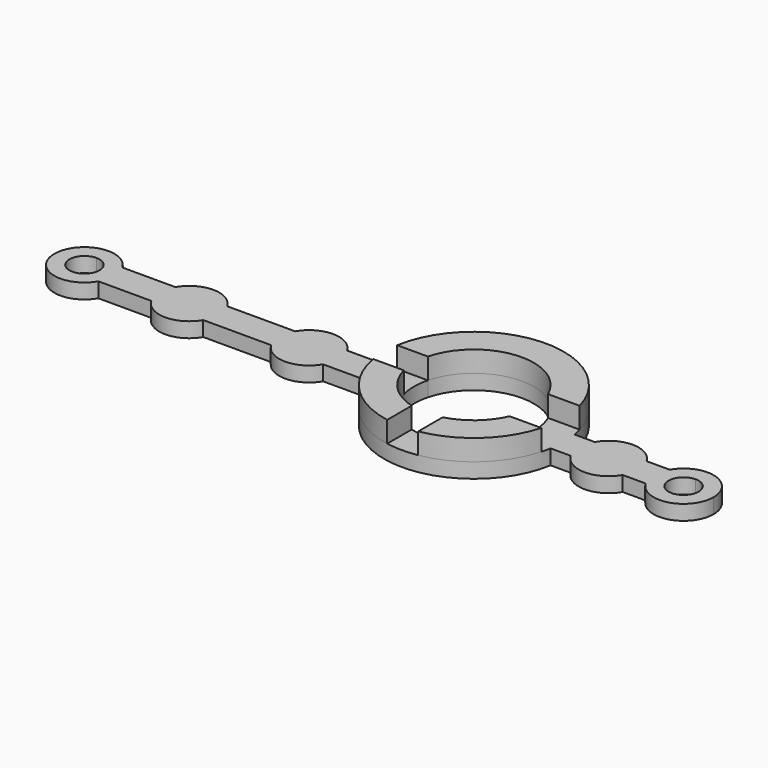
from build123d import *
from build123d import SkipClean  # not in build123d's __all__

# Parameters (mm, degrees)
F1_DEPTH = 5
F3_DEPTH = 7


with BuildPart() as f1:
    # F0 (on Top) → F1 (new body)
    with BuildSketch(Plane.XY):
        with BuildLine():
            ThreePointArc((0, 5), (3.5355339059, 3.5355339059), (5, 0))
            ThreePointArc((5, 0), (3.5355339059, -3.5355339059), (0, -5))
            Line((0, -5), (-8.6602540378, -5))
            ThreePointArc((-8.6602540378, -5), (2.588190451, -9.6592582629), (10, 0))
            ThreePointArc((10, 0), (2.588190451, 9.6592582629), (-8.6602540378, 5))
            Line((-8.6602540378, 5), (0, 5))
        make_face()
        with BuildLine():
            ThreePointArc((0, -5), (-5, 0), (0, 5))
            Line((0, 5), (-8.6602540378, 5))
            ThreePointArc((-8.6602540378, 5), (-10, 0), (-8.6602540378, -5))
            Line((-8.6602540378, -5), (0, -5))
        make_face()
        with BuildLine():
            ThreePointArc((-8.6602540378, -5), (-10, 0), (-8.6602540378, 5))
            Line((-8.6602540378, 5), (-16.3397459622, 5))
            ThreePointArc((-16.3397459622, 5), (-15.3407417371, 2.588190451), (-15, 0))
            ThreePointArc((-15, 0), (-15.3407417371, -2.588190451), (-16.3397459622, -5))
            Line((-16.3397459622, -5), (-8.6602540378, -5))
        make_face()
        with BuildLine():
            ThreePointArc((-15, 0), (-15.3407417371, 2.588190451), (-16.3397459622, 5))
            Line((-16.3397459622, 5), (-33.6602540378, 5))
            ThreePointArc((-33.6602540378, 5), (-35, 0), (-33.6602540378, -5))
            Line((-33.6602540378, -5), (-16.3397459622, -5))
            ThreePointArc((-16.3397459622, -5), (-15.3407417371, -2.588190451), (-15, 0))
        make_face()
        with BuildLine():
            Line((-33.6602540378, 5), (-16.3397459622, 5))
            ThreePointArc((-16.3397459622, 5), (-25, 10), (-33.6602540378, 5))
        make_face()
        with BuildLine():
            ThreePointArc((-33.6602540378, -5), (-25, -10), (-16.3397459622, -5))
            Line((-16.3397459622, -5), (-33.6602540378, -5))
        make_face()
        with BuildLine():
            ThreePointArc((-33.6602540378, -5), (-35, 0), (-33.6602540378, 5))
            Line((-33.6602540378, 5), (-40.4196010845, 5))
            ThreePointArc((-40.4196010845, 5), (-40.1050843164, 2.5087878084), (-40, 0))
            ThreePointArc((-40, 0), (-40.1050843164, -2.5087878084), (-40.4196010845, -5))
            Line((-40.4196010845, -5), (-33.6602540378, -5))
        make_face()
        with BuildLine():
            ThreePointArc((-40, 0), (-40.1050843164, 2.5087878084), (-40.4196010845, 5))
            Line((-40.4196010845, 5), (-50.635083269, 5))
            ThreePointArc((-50.635083269, 5), (-50.1594060747, 2.5200858497), (-50, 0))
            ThreePointArc((-50, 0), (-50.1594060747, -2.5200858497), (-50.635083269, -5))
            Line((-50.635083269, -5), (-40.4196010845, -5))
            ThreePointArc((-40.4196010845, -5), (-40.1050843164, -2.5087878084), (-40, 0))
        make_face()
        with BuildLine():
            Line((-50.635083269, 5), (-40.4196010845, 5))
            ThreePointArc((-40.4196010845, 5), (-70, 30), (-99.5803989155, 5))
            Line((-99.5803989155, 5), (-89.364916731, 5))
            ThreePointArc((-89.364916731, 5), (-70, 20), (-50.635083269, 5))
        make_face()
        with BuildLine():
            ThreePointArc((-99.5803989155, -5), (-70, -30), (-40.4196010845, -5))
            Line((-40.4196010845, -5), (-50.635083269, -5))
            ThreePointArc((-50.635083269, -5), (-70, -20), (-89.364916731, -5))
            Line((-89.364916731, -5), (-99.5803989155, -5))
        make_face()
        with BuildLine():
            ThreePointArc((-99.5803989155, -5), (-100, 0), (-99.5803989155, 5))
            Line((-99.5803989155, 5), (-116.3397459622, 5))
            ThreePointArc((-116.3397459622, 5), (-115.3407417371, 2.588190451), (-115, 0))
            ThreePointArc((-115, 0), (-115.3407417371, -2.588190451), (-116.3397459622, -5))
            Line((-116.3397459622, -5), (-99.5803989155, -5))
        make_face()
        with BuildLine():
            Line((-89.364916731, 5), (-99.5803989155, 5))
            ThreePointArc((-99.5803989155, 5), (-100, 0), (-99.5803989155, -5))
            Line((-99.5803989155, -5), (-89.364916731, -5))
            ThreePointArc((-89.364916731, -5), (-90, 0), (-89.364916731, 5))
        make_face()
        with BuildLine():
            ThreePointArc((-115, 0), (-115.3407417371, 2.588190451), (-116.3397459622, 5))
            Line((-116.3397459622, 5), (-133.6602540378, 5))
            ThreePointArc((-133.6602540378, 5), (-135, 0), (-133.6602540378, -5))
            Line((-133.6602540378, -5), (-116.3397459622, -5))
            ThreePointArc((-116.3397459622, -5), (-115.3407417371, -2.588190451), (-115, 0))
        make_face()
        with BuildLine():
            Line((-133.6602540378, 5), (-116.3397459622, 5))
            ThreePointArc((-116.3397459622, 5), (-125, 10), (-133.6602540378, 5))
        make_face()
        with BuildLine():
            ThreePointArc((-133.6602540378, -5), (-125, -10), (-116.3397459622, -5))
            Line((-116.3397459622, -5), (-133.6602540378, -5))
        make_face()
        with BuildLine():
            ThreePointArc((-133.6602540378, -5), (-135, 0), (-133.6602540378, 5))
            Line((-133.6602540378, 5), (-156.3397459622, 5))
            ThreePointArc((-156.3397459622, 5), (-155.3407417371, 2.588190451), (-155, 0))
            ThreePointArc((-155, 0), (-155.3407417371, -2.588190451), (-156.3397459622, -5))
            Line((-156.3397459622, -5), (-133.6602540378, -5))
        make_face()
        with BuildLine():
            ThreePointArc((-155, 0), (-155.3407417371, 2.588190451), (-156.3397459622, 5))
            Line((-156.3397459622, 5), (-173.6602540378, 5))
            ThreePointArc((-173.6602540378, 5), (-175, 0), (-173.6602540378, -5))
            Line((-173.6602540378, -5), (-156.3397459622, -5))
            ThreePointArc((-156.3397459622, -5), (-155.3407417371, -2.588190451), (-155, 0))
        make_face()
        with BuildLine():
            Line((-173.6602540378, 5), (-156.3397459622, 5))
            ThreePointArc((-156.3397459622, 5), (-165, 10), (-173.6602540378, 5))
        make_face()
        with BuildLine():
            ThreePointArc((-173.6602540378, -5), (-165, -10), (-156.3397459622, -5))
            Line((-156.3397459622, -5), (-173.6602540378, -5))
        make_face()
        with BuildLine():
            ThreePointArc((-173.6602540378, -5), (-175, 0), (-173.6602540378, 5))
            Line((-173.6602540378, 5), (-191.3397459622, 5))
            ThreePointArc((-191.3397459622, 5), (-190.3407417371, 2.588190451), (-190, 0))
            ThreePointArc((-190, 0), (-190.3407417371, -2.588190451), (-191.3397459622, -5))
            Line((-191.3397459622, -5), (-173.6602540378, -5))
        make_face()
        with BuildLine():
            ThreePointArc((-190, 0), (-190.3407417371, 2.588190451), (-191.3397459622, 5))
            Line((-191.3397459622, 5), (-200, 5))
            ThreePointArc((-200, 5), (-196.4644660941, 3.5355339059), (-195, 0))
            ThreePointArc((-195, 0), (-196.4644660941, -3.5355339059), (-200, -5))
            Line((-200, -5), (-191.3397459622, -5))
            ThreePointArc((-191.3397459622, -5), (-190.3407417371, -2.588190451), (-190, 0))
        make_face()
        with BuildLine():
            Line((-200, 5), (-191.3397459622, 5))
            ThreePointArc((-191.3397459622, 5), (-210, 0), (-191.3397459622, -5))
            Line((-191.3397459622, -5), (-200, -5))
            ThreePointArc((-200, -5), (-205, 0), (-200, 5))
        make_face()
    extrude(amount=F1_DEPTH)

    # F2 (on face) → F3 (join)
    with BuildSketch(Plane.XY.offset(5)):
        with BuildLine():
            ThreePointArc((-75.3128379583, -19.2814354452), (-84.2561475764, -14.0271970215), (-89.364916731, -5))
            Line((-89.364916731, -5), (-99.5803989155, -5))
            ThreePointArc((-99.5803989155, -5), (-91.3251821922, -21.1006304282), (-75.3128379583, -29.5258150239))
            Line((-75.3128379583, -29.5258150239), (-75.3128379583, -19.2814354452))
        make_face()
        with BuildLine():
            ThreePointArc((-41.0863354104, 8), (-71.5365980819, 29.9606219284), (-99.5803989155, 5))
            Line((-99.5803989155, 5), (-89.364916731, 5))
            ThreePointArc((-89.364916731, 5), (-71.5866967281, 19.9369604878), (-51.6696972202, 8))
            Line((-51.6696972202, 8), (-41.0863354104, 8))
        make_face()
        with BuildLine():
            ThreePointArc((-64.9254471064, -29.5677005012), (-49.8731234875, -22.2465467399), (-41.0863354104, -8))
            Line((-41.0863354104, -8), (-51.6696972202, -8))
            ThreePointArc((-51.6696972202, -8), (-56.9951167094, -15.1945059346), (-64.9254471064, -19.345514026))
            Line((-64.9254471064, -19.345514026), (-64.9254471064, -29.5677005012))
        make_face()
    with SkipClean():  # cleaning this boolean's faces spoils the solid; the shape is the same uncleaned
        extrude(amount=F3_DEPTH)


solid = f1.part
